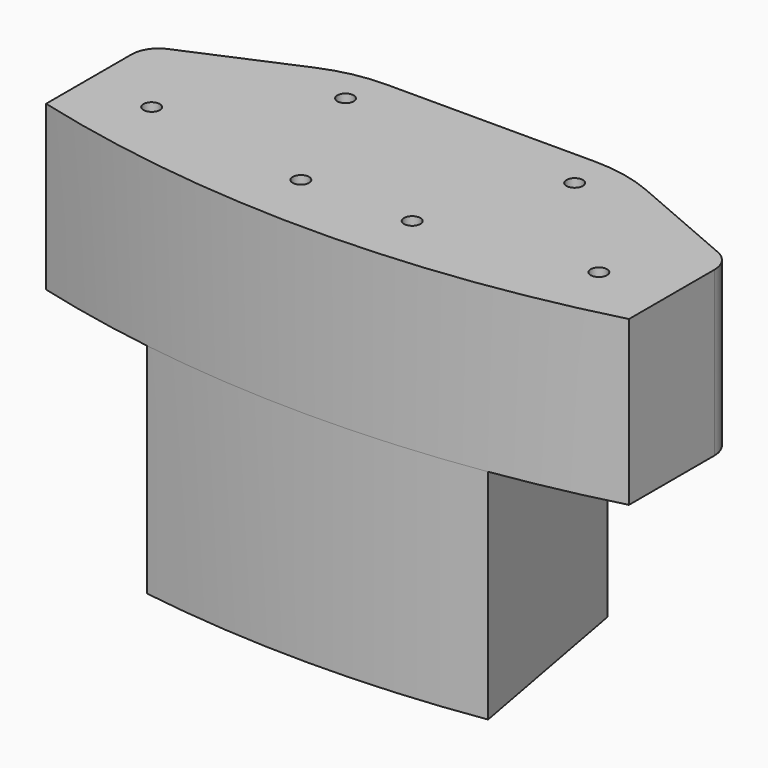
from build123d import *

# Parameters (mm, degrees)
F1_DEPTH = 30
F2_R     = 1.5
F3_DEPTH = 30.001
F4_R     = 28.5239911769
F5_R     = 5
F7_R     = 1.5
F8_DEPTH = 40


with BuildPart() as f1:
    # F0 (on Top) → F1 (new body)
    with BuildSketch(Plane.XY):
        with BuildLine():
            Line((-53.4347956585, -180.2462832153), (-53.4347956585, -203.0879676715))
            ThreePointArc((-53.4347956585, -203.0879676715), (0, -210), (53.4347956585, -203.0879676715))
            Line((53.4347956585, -203.0879676715), (53.4347956585, -180.2462832153))
            Line((53.4347956585, -180.2462832153), (25, -168))
            Line((25, -168), (0, -168))
            Line((0, -168), (-25, -168))
            Line((-25, -168), (-53.4347956585, -180.2462832153))
        make_face()
    extrude(amount=F1_DEPTH)

    # F2 (on face) → F3 (cut, through all)
    with BuildSketch(Plane.XY.offset(30)):
        with Locations((-61.4929363222, -189.1117421473)):
            Circle(F2_R)
        with Locations((-116.9707156809, -160.8515617902)):
            Circle(F2_R)
        with Locations((-161.0003432552, -116.8309564779)):
            Circle(F2_R)
        with Locations((-189.2718923255, -61.3589697679)):
            Circle(F2_R)
        with Locations((-199.0179466895, 0.1344137845)):
            Circle(F2_R)
        with Locations((61.4958267934, -189.0991398316)):
            Circle(F2_R)
        with Locations((116.9678135034, -160.8275907612)):
            Circle(F2_R)
        with Locations((160.9884188157, -116.7979631869)):
            Circle(F2_R)
        with Locations((189.2485991728, -61.3201838282)):
            Circle(F2_R)
        with Locations((198.9820512211, 0.175195735)):
            Circle(F2_R)
        with Locations((-20.9999999994, -175.0021517963)):
            Circle(F2_R)
        with Locations((-40.9903269079, -194.4499816389)):
            Circle(F2_R)
        with Locations((-10.2028351662, -198.7382755147)):
            Circle(F2_R)
        with Locations((20.9999997802, -174.9978481734)):
            Circle(F2_R)
        with Locations((10.2076995225, -198.7361841041)):
            Circle(F2_R)
        with Locations((40.9943117987, -194.4415809015)):
            Circle(F2_R)
    extrude(amount=-F3_DEPTH, mode=Mode.SUBTRACT)

    # F4
    f4_edges = [f1.edges().sort_by_distance(p)[0] for p in [
        (25, -168, 15),
        (-25, -168, 15),
    ]]
    fillet(f4_edges, radius=F4_R)

    # F5
    f5_edges = [f1.edges().sort_by_distance(p)[0] for p in [
        (53.434796, -180.246283, 15),
        (-53.434796, -180.246283, 15),
    ]]
    fillet(f5_edges, radius=F5_R)

    # F7 (on face) → F8 (join)
    with BuildSketch(Plane(origin=(0, 0, 0), x_dir=(1, 0, 0), z_dir=(0, 0, -1))):
        with BuildLine():
            ThreePointArc((31.2604393052, 207.6602632533), (0, 210), (-31.2604393052, 207.6602632533))
            Line((-31.2604393052, 207.6602632533), (-24.7243543685, 172.0646172762))
            Line((-24.7243543685, 172.0646172762), (0, 172.0646172762))
            Line((0, 172.0646172762), (24.7243543685, 172.0646172762))
            Line((24.7243543685, 172.0646172762), (31.2604393052, 207.6602632533))
        make_face()
        with Locations((-20.9999999994, 175.0021517963)):
            Circle(F7_R, mode=Mode.SUBTRACT)
        with Locations((20.9999997802, 174.9978481734)):
            Circle(F7_R, mode=Mode.SUBTRACT)
        with Locations((-10.2028351662, 198.7382755147)):
            Circle(F7_R, mode=Mode.SUBTRACT)
        with Locations((10.2076995225, 198.7361841041)):
            Circle(F7_R, mode=Mode.SUBTRACT)
    extrude(amount=F8_DEPTH)


solid = f1.part
